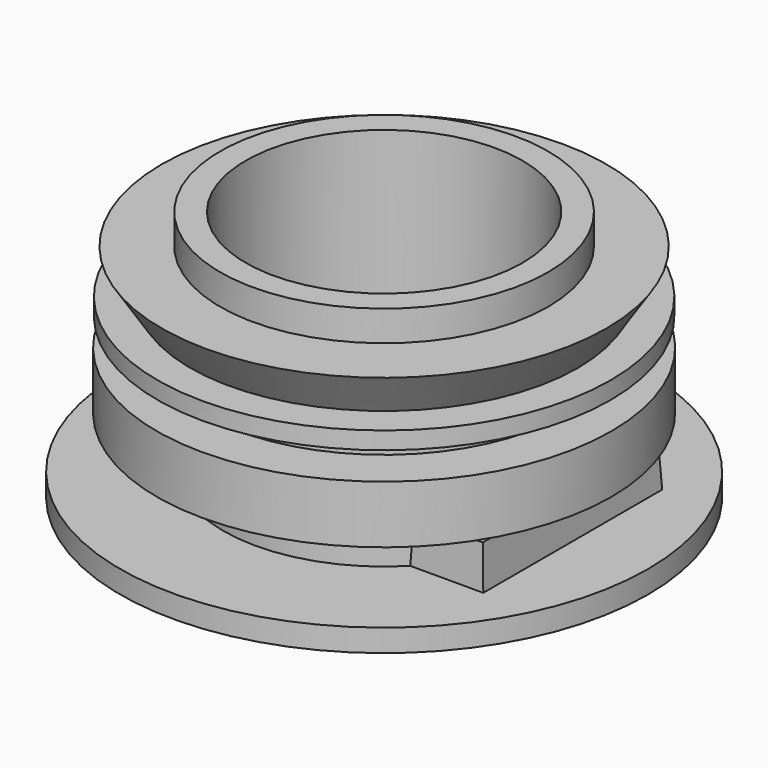
from build123d import *

# Parameters (mm, degrees)
F0_W     = 67.9279565811
F0_H     = 88.0647003651
F1_DEPTH = 25.4
F1_TAPER = 3


# Not quite as in the source:
# - a feature of the source that left no trace in its solid (it failed there, or was rolled back) is left out


with BuildPart() as f1:
    # F0 (on Top) → F1 (new body)
    with BuildSketch(Plane.XY):
        Rectangle(F0_W, F0_H)
    extrude(amount=F1_DEPTH, taper=F1_TAPER)

    # F2 (on Front) → F3 (revolve)
    with BuildSketch(Plane.XZ):
        Polygon((13.9438202605, 97.8820249438), (13.9438202605, 0), (62.8700107336, 0), (62.8700107336, 8.7491702288), (22.6633418351, 8.7491702288), (22.6633418351, 28.8525056094), (48.57968539, 28.8525056094), (48.57968539, 51.3779297471), (30.8984406292, 51.3779297471), (30.8984406292, 63.9727860689), (48.3374781907, 62.0351172984), (48.3374781907, 68.8169673085), (35.5004072189, 68.8169673085), (46.6420166194, 86.0137939453), (23.8743834198, 86.0137939453), (23.8743834198, 97.8820249438), align=None)
    revolve(axis=Axis((-40, 0, 38.2511918375), (0, 0, 1)))


solid = f1.part
